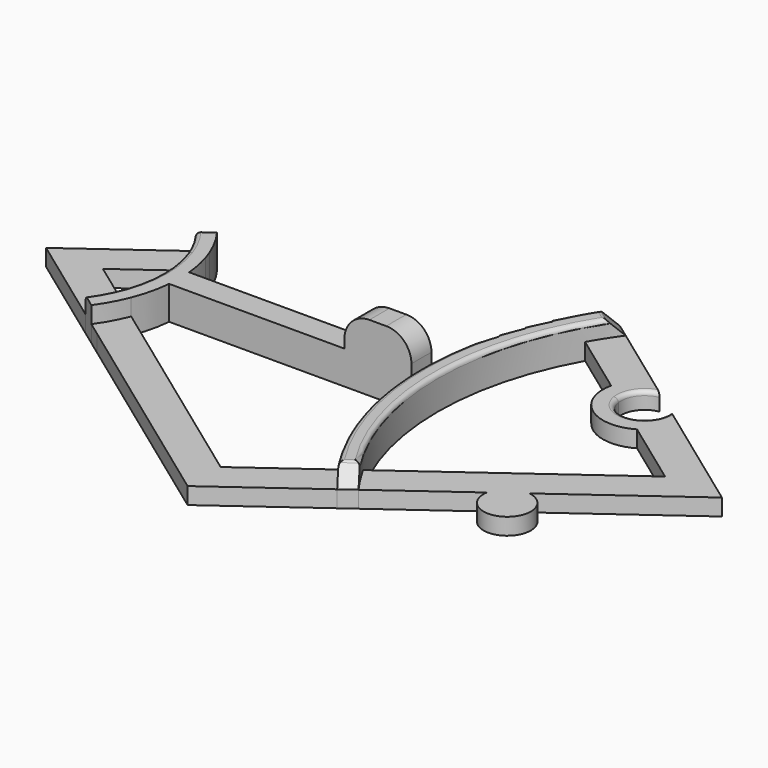
from build123d import *

# Parameters (mm, degrees)
F1_DEPTH = 2
F2_R     = 0.5
F3_DEPTH = 4
F4_SIZE  = 2
F5_R     = 0.5
F6_DEPTH = 8
F7_R     = 3


# Not quite as in the source:
# - a feature names something its author has since deleted; it is built from what else it names


with BuildPart() as f1:
    # F0 (on Top) → F1 (new body)
    with BuildSketch(Plane.XY):
        with BuildLine():
            Line((25.88854382, -10.5801345413), (40.4508497187, 0))
            Line((40.4508497187, 0), (25.88854382, 10.5801345413))
            ThreePointArc((25.88854382, 10.5801345413), (25.3831849379, 8.475163306), (23.5374028108, 7.3440665638))
            Line((23.5374028108, 7.3440665638), (25.6267504373, 5.8260666573))
            Line((25.6267504373, 5.8260666573), (33.6456432519, 0))
            Line((33.6456432519, 0), (10.7841511133, -16.6098462924))
            ThreePointArc((10.7841511133, -16.6098462924), (11.814451709, -18.3291218838), (12.94427191, -19.9846985779))
            Line((12.94427191, -19.9846985779), (22.6524758425, -12.9312755504))
            Line((22.6524758425, -12.9312755504), (25.88854382, -10.5801345413))
        make_face()
        with BuildLine():
            ThreePointArc((22.6524758425, -12.9312755504), (27.1085880869, -15.6619846459), (25.88854382, -10.5801345413))
            Line((25.88854382, -10.5801345413), (22.6524758425, -12.9312755504))
        make_face()
        with BuildLine():
            Line((25.6267504373, 5.8260666573), (23.5374028108, 7.3440665638))
            ThreePointArc((23.5374028108, 7.3440665638), (21.4324315756, 7.8494254458), (20.3013348333, 9.6952075729))
            Line((20.3013348333, 9.6952075729), (18.2119872068, 11.2132074794))
            ThreePointArc((18.2119872068, 11.2132074794), (20.1560130652, 6.0925860852), (25.6267504373, 5.8260666573))
        make_face()
        with BuildLine():
            Line((18.2119872068, 11.2132074794), (20.3013348333, 9.6952075729))
            ThreePointArc((20.3013348333, 9.6952075729), (20.8066937154, 11.8001788082), (22.6524758425, 12.9312755504))
            Line((22.6524758425, 12.9312755504), (12.94427191, 19.9846985779))
            ThreePointArc((12.94427191, 19.9846985779), (11.814451709, 18.3291218838), (10.7841511133, 16.6098462924))
            Line((10.7841511133, 16.6098462924), (18.2119872068, 11.2132074794))
        make_face()
    extrude(amount=F1_DEPTH)

    # F2
    f2_edges = [f1.edges().sort_by_distance(p)[0] for p in [
        (21.432432, 7.849425, 2),
    ]]
    fillet(f2_edges, radius=F2_R)



with BuildPart() as f1b:
    # F0 (on Top) → F1, piece 2 (new body)
    with BuildSketch(Plane.XY):
        with BuildLine():
            Line((0, -29.3892626146), (11.3262379212, -21.1602690825))
            ThreePointArc((11.3262379212, -21.1602690825), (10.1939633159, -19.506943), (9.1554367996, -17.7931765073))
            Line((9.1554367996, -17.7931765073), (0, -24.4449907046))
            Line((0, -24.4449907046), (-25.5664713255, -5.8698619956))
            ThreePointArc((-25.5664713255, -5.8698619956), (-26.4247321499, -7.6985729811), (-27.5065778087, -9.4045640367))
            Line((-27.5065778087, -9.4045640367), (-25.88854382, -10.5801345413))
            Line((-25.88854382, -10.5801345413), (-14.5623058987, -18.8091280734))
            Line((-14.5623058987, -18.8091280734), (0, -29.3892626146))
        make_face()
    extrude(amount=F1_DEPTH)


with BuildPart() as f1c:
    # F0 (on Top) → F1, piece 3 (new body)
    with BuildSketch(Plane.XY):
        with BuildLine():
            Line((9.1554367996, -17.7931765073), (10.7841511133, -16.6098462924))
            ThreePointArc((10.7841511133, -16.6098462924), (6.4508497187, 0), (10.7841511133, 16.6098462924))
            Line((10.7841511133, 16.6098462924), (9.1554367996, 17.7931765073))
            ThreePointArc((9.1554367996, 17.7931765073), (5.8461773909, 9.9255555553), (4.4821132939, 1.5))
            ThreePointArc((4.4821132939, 1.5), (4.4508497187, 0), (4.4821132939, -1.5))
            ThreePointArc((4.4821132939, -1.5), (5.8461773909, -9.9255555553), (9.1554367996, -17.7931765073))
        make_face()
    extrude(amount=F1_DEPTH)


with BuildPart() as f1d:
    # F0 (on Top) → F1, piece 4 (new body)
    with BuildSketch(Plane.XY):
        with BuildLine():
            ThreePointArc((-29.1246117975, -8.2289935321), (-28.0552509558, -6.5076210175), (-27.2456067433, -4.6498987043))
            Line((-27.2456067433, -4.6498987043), (-33.6456432519, 0))
            Line((-33.6456432519, 0), (-27.2456067433, 4.6498987043))
            ThreePointArc((-27.2456067433, 4.6498987043), (-28.0552509558, 6.5076210175), (-29.1246117975, 8.2289935321))
            Line((-29.1246117975, 8.2289935321), (-40.4508497187, 0))
            Line((-40.4508497187, 0), (-29.1246117975, -8.2289935321))
        make_face()
    extrude(amount=F1_DEPTH)


with BuildPart() as f1_1:
    add(f1.part)

    add(f1b.part)  # F3 merges F1b

    add(f1c.part)  # F3 merges F1c

    add(f1d.part)  # F3 merges F1d
    # F0 (on Top) → F3 (join)
    with BuildSketch(Plane.XY):
        with BuildLine():
            Line((-27.2456067433, -4.6498987043), (-25.5664713255, -5.8698619956))
            ThreePointArc((-25.5664713255, -5.8698619956), (-24.8897380342, -3.7218010616), (-24.5213173967, -1.5))
            ThreePointArc((-24.5213173967, -1.5), (-24.4508497187, 0), (-24.5213173967, 1.5))
            ThreePointArc((-24.5213173967, 1.5), (-24.7650379905, 3.1552037061), (-25.1802669457, 4.7759084761))
            ThreePointArc((-25.1802669457, 4.7759084761), (-25.3634508604, 5.3263867387), (-25.5664713255, 5.8698619956))
            Line((-25.5664713255, 5.8698619956), (-27.2456067433, 4.6498987043))
            ThreePointArc((-27.2456067433, 4.6498987043), (-26.4508497187, 0), (-27.2456067433, -4.6498987043))
        make_face()
        with BuildLine():
            Line((9.1554367996, -17.7931765073), (10.7841511133, -16.6098462924))
            ThreePointArc((10.7841511133, -16.6098462924), (6.4508497187, 0), (10.7841511133, 16.6098462924))
            Line((10.7841511133, 16.6098462924), (9.1554367996, 17.7931765073))
            ThreePointArc((9.1554367996, 17.7931765073), (5.8461773909, 9.9255555553), (4.4821132939, 1.5))
            ThreePointArc((4.4821132939, 1.5), (4.4508497187, 0), (4.4821132939, -1.5))
            ThreePointArc((4.4821132939, -1.5), (5.8461773909, -9.9255555553), (9.1554367996, -17.7931765073))
        make_face()
        with BuildLine():
            Line((11.3262379212, -21.1602690825), (12.94427191, -19.9846985779))
            ThreePointArc((12.94427191, -19.9846985779), (11.814451709, -18.3291218838), (10.7841511133, -16.6098462924))
            Line((10.7841511133, -16.6098462924), (9.1554367996, -17.7931765073))
            ThreePointArc((9.1554367996, -17.7931765073), (10.1939633159, -19.506943), (11.3262379212, -21.1602690825))
        make_face()
        with BuildLine():
            Line((9.1554367996, 17.7931765073), (10.7841511133, 16.6098462924))
            ThreePointArc((10.7841511133, 16.6098462924), (11.814451709, 18.3291218838), (12.94427191, 19.9846985779))
            Line((12.94427191, 19.9846985779), (11.3262379212, 21.1602690825))
            ThreePointArc((11.3262379212, 21.1602690825), (10.1939633159, 19.506943), (9.1554367996, 17.7931765073))
        make_face()
        with BuildLine():
            Line((-24.5213173967, -1.5), (-3.5491502813, -1.5))
            Line((-3.5491502813, -1.5), (-3.5491502813, 1.5))
            Line((-3.5491502813, 1.5), (-24.5213173967, 1.5))
            ThreePointArc((-24.5213173967, 1.5), (-24.4508497187, 0), (-24.5213173967, -1.5))
        make_face()
        with BuildLine():
            ThreePointArc((-27.5065778087, -9.4045640367), (-26.4247321499, -7.6985729811), (-25.5664713255, -5.8698619956))
            Line((-25.5664713255, -5.8698619956), (-27.2456067433, -4.6498987043))
            ThreePointArc((-27.2456067433, -4.6498987043), (-28.0552509558, -6.5076210175), (-29.1246117975, -8.2289935321))
            Line((-29.1246117975, -8.2289935321), (-27.5065778087, -9.4045640367))
        make_face()
        with BuildLine():
            ThreePointArc((-25.5664713255, 5.8698619956), (-26.4247321499, 7.6985729811), (-27.5065778087, 9.4045640367))
            Line((-27.5065778087, 9.4045640367), (-29.1246117975, 8.2289935321))
            ThreePointArc((-29.1246117975, 8.2289935321), (-28.0552509558, 6.5076210175), (-27.2456067433, 4.6498987043))
            Line((-27.2456067433, 4.6498987043), (-25.5664713255, 5.8698619956))
        make_face()
    extrude(amount=F3_DEPTH)

    # F4
    f4_edges = [f1_1.edges().sort_by_distance(p)[0] for p in [
        (12.135255, 20.572484, 4),
        (12.135255, -20.572484, 4),
    ]]
    chamfer(f4_edges, length=F4_SIZE)

    # F5
    f5_edges = [f1_1.edges().sort_by_distance(p)[0] for p in [
        (-26.45085, 0, 4),
        (11.00599, 18.920807, 4),
        (4.45085, 0, 4),
        (6.45085, 0, 4),
        (11.00599, -18.920807, 4),
    ]]
    fillet(f5_edges, radius=F5_R)

    # F0 (on Top) → F6 (join)
    with BuildSketch(Plane.XY):
        with BuildLine():
            Line((-3.5491502813, -1.5), (4.4821132939, -1.5))
            ThreePointArc((4.4821132939, -1.5), (4.4508497187, 0), (4.4821132939, 1.5))
            Line((4.4821132939, 1.5), (-3.5491502813, 1.5))
            Line((-3.5491502813, 1.5), (-3.5491502813, -1.5))
        make_face()
    extrude(amount=F6_DEPTH)

    # F7
    f7_edges = [f1_1.edges().sort_by_distance(p)[0] for p in [
        (4.45085, 0, 8),
        (-3.54915, 0, 8),
    ]]
    fillet(f7_edges, radius=F7_R)


solid = f1_1.part
